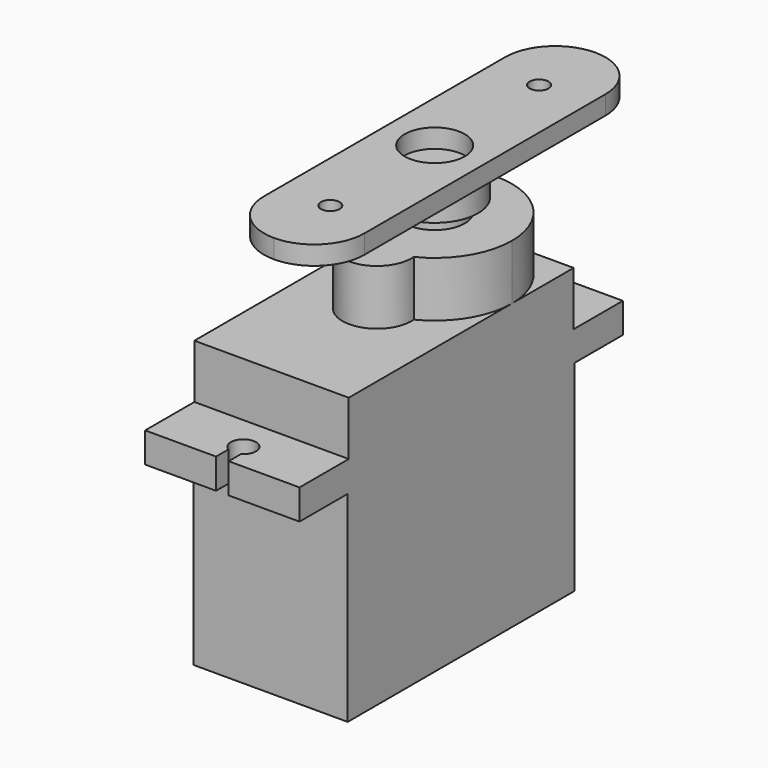
from build123d import *

# Parameters (mm, degrees)
F1_DEPTH  = 2.4
F2_W      = 12.3
F2_H      = 22.4
F3_DEPTH  = 4.3
F5_DEPTH  = 4.4
F6_W      = 12.3
F6_H      = 22.6
F7_DEPTH  = 16
F8_R      = 2.4
F9_DEPTH  = 3.2
F10_W     = 8
F10_H     = 32
F10_R     = 0.75
F10_R_2   = 2.4
F11_DEPTH = 1.5
F12_R     = 3.45
F12_R_2   = 2.4
F13_DEPTH = 2.15
F14_R     = 3.99999


# Not quite as in the source:
# - a fillet or chamfer is up to 0.001 mm smaller than in the source, because OpenCascade refuses the exact size


with BuildPart() as f1:
    # F0 (on Top) → F1 (new body)
    with BuildSketch(Plane.XY):
        with BuildLine():
            Line((0.5, -16.1), (6.15, -16.1))
            Line((6.15, -16.1), (6.15, 16.1))
            Line((6.15, 16.1), (0.5, 16.1))
            Line((0.5, 16.1), (0.5, 14.8660254038))
            ThreePointArc((0.5, 14.8660254038), (0, 13), (-0.5, 14.8660254038))
            Line((-0.5, 14.8660254038), (-0.5, 16.1))
            Line((-0.5, 16.1), (-6.15, 16.1))
            Line((-6.15, 16.1), (-6.15, -16.1))
            Line((-6.15, -16.1), (-0.5, -16.1))
            Line((-0.5, -16.1), (-0.5, -14.8660254038))
            ThreePointArc((-0.5, -14.8660254038), (0, -13), (0.5, -14.8660254038))
            Line((0.5, -14.8660254038), (0.5, -16.1))
        make_face()
    extrude(amount=F1_DEPTH)

    # F2 (on face) → F3 (join)
    with BuildSketch(Plane.XY.offset(2.4)):
        Rectangle(F2_W, F2_H)
    extrude(amount=F3_DEPTH)

    # F4 (on face) → F5 (join)
    with BuildSketch(Plane.XY.offset(6.7)):
        with BuildLine():
            ThreePointArc((-6.15, 5.0500000209), (-5.2282149501, 1.8114403764), (-2.7391809778, -0.4563043478))
            ThreePointArc((-2.7391809778, -0.4563043478), (0, -3.45), (2.7391809778, -0.4563043478))
            ThreePointArc((2.7391809778, -0.4563043478), (5.2282149446, 1.8114403675), (6.15, 5.05))
            ThreePointArc((6.15, 5.05), (4.3487067043, 9.3987067043), (0, 11.2))
            ThreePointArc((0, 11.2), (-4.3487066969, 9.3987067117), (-6.15, 5.0500000209))
        make_face()
    extrude(amount=F5_DEPTH)

    # F6 (on face) → F7 (join)
    with BuildSketch(Plane(origin=(0, 0, 0), x_dir=(1, 0, 0), z_dir=(0, 0, -1))):
        Rectangle(F6_W, F6_H)
    extrude(amount=F7_DEPTH)


with BuildPart() as f9:
    # F8 (on face) → F9 (new body)
    with BuildSketch(Plane.XY.offset(11.1)):
        with Locations((0, 5.05)):
            Circle(F8_R)
    extrude(amount=F9_DEPTH)


with BuildPart() as f11:
    # F10 (on face) → F11 (new body)
    with BuildSketch(Plane.XY.offset(14.3)):
        with Locations((0, 5.05)):
            Rectangle(F10_W, F10_H)
        with Locations((0, -5.35)):
            Circle(F10_R, mode=Mode.SUBTRACT)
        with Locations((0, 5.05)):
            Circle(F10_R_2, mode=Mode.SUBTRACT)
        with Locations((0, 15.45)):
            Circle(F10_R, mode=Mode.SUBTRACT)
    extrude(amount=F11_DEPTH)

    # F12 (on face) → F13 (join)
    with BuildSketch(Plane(origin=(0, 0, 14.3), x_dir=(1, 0, 0), z_dir=(0, 0, -1))):
        with Locations((0, -5.05)):
            Circle(F12_R)
        with Locations((0, -5.05)):
            Circle(F12_R_2, mode=Mode.SUBTRACT)
    extrude(amount=F13_DEPTH)

    # F14 (radius 4 in the source; OpenCascade refuses exactly that, so slightly less here)
    f14_edges = [f11.edges().sort_by_distance(p)[0] for p in [
        (4, 21.05, 15.05),
        (-4, 21.05, 15.05),
        (4, -10.95, 15.05),
        (-4, -10.95, 15.05),
    ]]
    fillet(f14_edges, radius=F14_R)


solid = Compound([f1.part, f9.part, f11.part])
